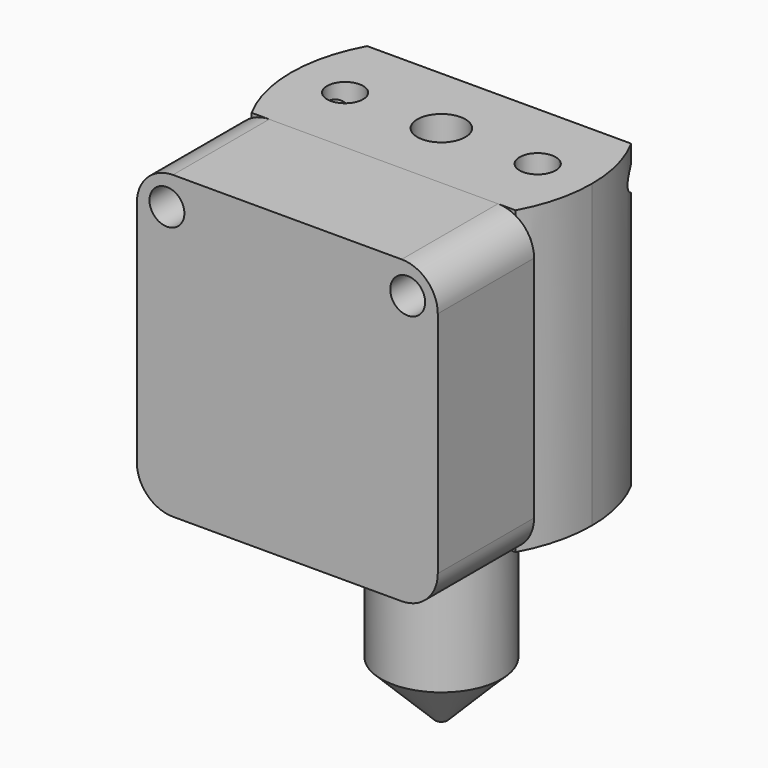
from build123d import *

# Parameters (mm, degrees)
F0_W     = 25
F0_H     = 25
F1_DEPTH = 6
F4_R     = 26.2066514647
F4_R_2   = 2
F4_R_3   = 1.5
F5_DEPTH = 25
F6_W     = 1.5341439003
F6_H     = 25
F6_W_2   = 21.9317121995
F7_DEPTH = 10
F8_R     = 1.45
F9_DEPTH = 25
F10_R    = 3


with BuildPart() as f1:
    # F0 (on Front) → F1 (new body, symmetric)
    with BuildSketch(Plane.XZ):
        with Locations((0, -12.5)):
            Rectangle(F0_W, F0_H)
    extrude(amount=F1_DEPTH, both=True)

    # F2 (on Front) → F3 (revolve)
    with BuildSketch(Plane.XZ):
        Polygon((5, -25), (0, -25), (0, -43.16), (0.5, -43.16), (5, -38.66), align=None)
    revolve(axis=Axis((0, 0, -34.08), (0, 0, -1)))

    # F4 (on face) → F5 (cut)
    with BuildSketch(Plane.XY):
        Circle(F4_R)
        with BuildLine():
            Line((12.5, 6), (12.5, 0))
            Line((12.5, 0), (12.5, -6))
            Line((12.5, -6), (10.9658560997, -6))
            ThreePointArc((10.9658560997, -6), (0, -12.5), (-10.9658560997, -6))
            Line((-10.9658560997, -6), (-12.5, -6))
            Line((-12.5, -6), (-12.5, 0))
            Line((-12.5, 0), (-12.5, 6))
            Line((-12.5, 6), (-10.9658560997, 6))
            ThreePointArc((-10.9658560997, 6), (0, 12.5), (10.9658560997, 6))
            Line((10.9658560997, 6), (12.5, 6))
        make_face(mode=Mode.SUBTRACT)
        Circle(F4_R_2)
        with Locations((-8, 0)):
            Circle(F4_R_3)
        with Locations((8, 0)):
            Circle(F4_R_3)
        with BuildLine():
            Line((12.5, -6), (12.5, 0))
            ThreePointArc((12.5, 0), (12.1103922572, -3.0965140685), (10.9658560997, -6))
            Line((10.9658560997, -6), (12.5, -6))
        make_face()
        with BuildLine():
            ThreePointArc((10.9658560997, 6), (12.1103922572, 3.0965140685), (12.5, 0))
            Line((12.5, 0), (12.5, 6))
            Line((12.5, 6), (10.9658560997, 6))
        make_face()
        with BuildLine():
            ThreePointArc((-12.5, 0), (-12.1103922572, 3.0965140685), (-10.9658560997, 6))
            Line((-10.9658560997, 6), (-12.5, 6))
            Line((-12.5, 6), (-12.5, 0))
        make_face()
        with BuildLine():
            Line((-12.5, -6), (-10.9658560997, -6))
            ThreePointArc((-10.9658560997, -6), (-12.1103922572, -3.0965140685), (-12.5, 0))
            Line((-12.5, 0), (-12.5, -6))
        make_face()
    extrude(amount=-F5_DEPTH, mode=Mode.SUBTRACT)


with BuildPart() as f7:
    # F6 (on face) → F7 (new body)
    with BuildSketch(Plane.XZ.offset(6)):
        with Locations((-11.7329280499, -12.5)):
            Rectangle(F6_W, F6_H)
        with Locations((0, -12.5)):
            Rectangle(F6_W_2, F6_H)
        with Locations((11.7329280499, -12.5)):
            Rectangle(F6_W, F6_H)
    extrude(amount=F7_DEPTH)


with BuildPart() as f9_tool:
    # F8 (on face) → F9 (new body)
    with BuildSketch(Plane.XZ.offset(16)):
        with Locations((-10, -2.5)):
            Circle(F8_R)
        with Locations((10, -2.5)):
            Circle(F8_R)
    extrude(amount=-F9_DEPTH)


with BuildPart() as f1_1:
    add(f1.part)

    # F9: cut by f9_tool
    add(f9_tool.part, mode=Mode.SUBTRACT)


with BuildPart() as f7_1:
    add(f7.part)

    # F9: cut by f9_tool
    add(f9_tool.part, mode=Mode.SUBTRACT)

    # F10
    f10_edges = [f7_1.edges().sort_by_distance(p)[0] for p in [
        (12.5, -11, 0),
        (-12.5, -11, 0),
        (-12.5, -11, -25),
        (12.5, -11, -25),
    ]]
    fillet(f10_edges, radius=F10_R)


solid = Compound([f1_1.part, f7_1.part])
